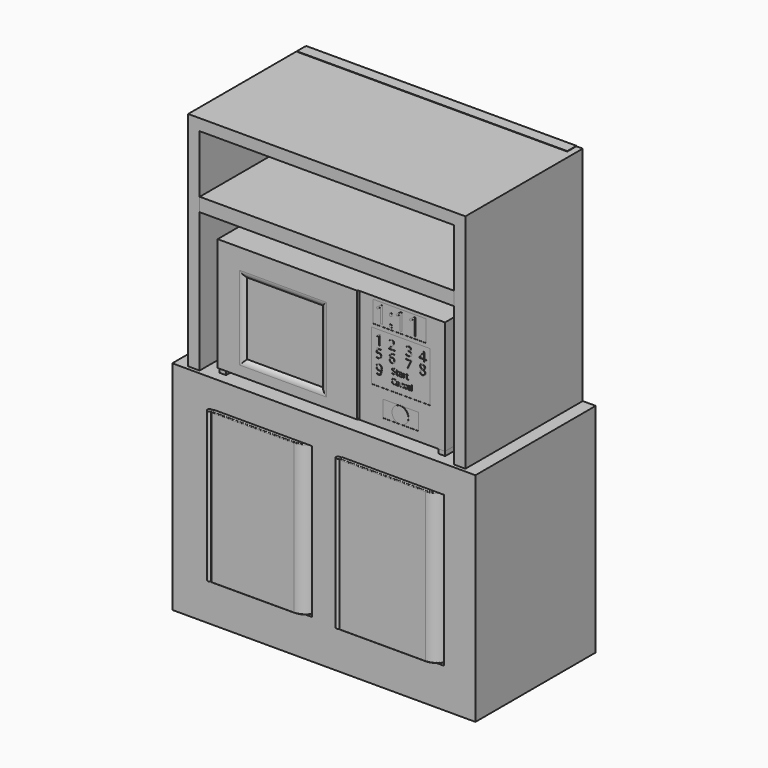
from build123d import *

# Parameters (mm, degrees)
F1_DEPTH        = 50.8
F2_DEPTH        = 52.07
F3_W            = 3.9822123945
F3_H            = 77.1151632071
F4_DEPTH        = 55.118
F5_DEPTH        = 38.354
F6_W            = 35.2624859661
F6_H            = 52.127157338
F6_W_2          = 33.9852
F7_DEPTH        = 43.18
F8_W            = 45.6940376786
F8_H            = 2.6725903153
F8_W_2          = 33.9852
F9_DEPTH        = 40.64
F10_R           = 2.8255137631
F11_DEPTH       = 25.4
F13_START       = 2.286
F12_W           = 78.4899894114
F12_H           = 39.2950200476
F12_R           = 2.8255137631
F13_DEPTH       = 42.418
F14_R           = 2.8255137631
F15_DEPTH       = 0.0762
F15_DEPTH_BACK  = 42.7228
F16_W           = 26.2017082423
F16_H           = 24.9313246459
F17_DEPTH       = 0.3048
F16_W_2         = 0.4919990897
F16_H_2         = 39.1533517959
F18_DEPTH       = 2.8702
F19_DEPTH       = 0.635
F20_T1_DEPTH    = 24.9313246459
F20_T3_DEPTH    = 26.2017082423
F20_T9_DEPTH    = 31.1330873344
F20_T13_DEPTH   = 29.862703738
F20_T20_DEPTH   = 29.862703738
F20_T24_DEPTH   = 31.1330873344
F20_T31_DEPTH   = 31.1330873344
F20_T35_DEPTH   = 29.862703738
F20_T42_DEPTH   = 31.1330873344
F20_T46_DEPTH   = 29.862703738
F21_W           = 18.2726848871
F21_H           = 7.4134916067
F21_W_2         = 20.2405880716
F21_H_2         = 17.3329468817
F21_W_3         = 12.3210083693
F21_H_3         = 5.7428432629
F21_R           = 2.8255137631
F15_FACE_R      = 2.8255137631
F22_DEPTH       = 0.0508
F23_TEXT_SIZE   = 4.6472272111
F23_TEXT_SIZE_2 = 4.3617124602
F23_TEXT_SIZE_3 = 4.3842428144
F23_TEXT_SIZE_4 = 2.6675458584
F23_TEXT_SIZE_5 = 2.4056812334
F23_TEXT_SIZE_6 = 4.3257706509
F23_TEXT_SIZE_7 = 4.6672040804
F23_TEXT_SIZE_8 = 4.7208482607
F24_DEPTH       = 0.127
F25_R           = 0.8497114132
F26_DEPTH       = 29.21
F27_W           = 33.685291186
F27_H           = 14.8179726675
F27_H_2         = 2.6725903153
F28_DEPTH       = 3.81
F27_W_2         = 34.7396545112
F27_H_3         = 52.0917661488
F29_DEPTH       = 3.81
F30_T1_DEPTH    = 76.6830152699
F30_2_T1_DEPTH  = 76.6852103972
F31_R           = 0.254
F31_2_R         = 0.254
F32_TEXT_SIZE   = 8.062650967
F33_DEPTH       = 0.0762
F35_START       = -9.652
F34_R           = 0.8068869831
F34_R_2         = 0.7608241077
F35_DEPTH       = 51.816
F37_DEPTH       = 2.1844
F38_R           = 0.1742456075
F38_W           = 0.127
F38_H           = 0.7986426353
F38_W_2         = 0.1268871129
F39_DEPTH       = 1.1684
F40_R           = 0.127
F41_R           = 0.0254
F42_W           = 2.2606
F42_H           = 1.7440778902
F42_W_2         = 2.2516623139
F42_H_2         = 1.757984166
F43_DEPTH       = 44.45
F44_W           = 88.0871986938
F44_H           = 4.7152489424
F45_DEPTH       = 46.7614


# Not quite as in the source:
# - a fillet or chamfer that OpenCascade refuses, or shapes differently, is made with other operations: its cross-section is extruded or revolved along the edge and cut away or added
# - a feature names something its author has since deleted; it is built from what else it names
# - Text() gives the source's letters only with a copy of the font that has no kerning and outlines rounded to 1/6400 em; it was checked with that copy


with BuildPart() as f1:
    # F0 (on Front) → F1 (new body)
    with BuildSketch(Plane.XZ):
        Polygon((57.3023967445, 76.9620016217), (-38.7095995247, 76.9620016217), (-38.7095995247, 0), (-34.7471995247, 0), (-34.7471995247, 72.9995965958), (53.3399991691, 72.9995965958), (53.3399991691, 0), (57.3023967445, 0), align=None)
    extrude(amount=F1_DEPTH)

    # F0 (on Front) → F2 (join)
    with BuildSketch(Plane.XZ):
        Polygon((-34.7471995247, 0), (-38.7095995247, 0), (-43.196324259, 0), (-43.196324259, -75.2101317048), (61.7981967445, -75.2101317048), (61.7981967445, 0), (57.3023967445, 0), (53.3399991691, 0), align=None)
    extrude(amount=F2_DEPTH)

    # F3 (on Right) → F4 (join)
    with BuildSketch(Plane.YZ):
        with Locations((-1.9911061972, 38.5575816035)):
            Rectangle(F3_W, F3_H)
    extrude(amount=F4_DEPTH)

    # F3 (on Right) → F5 (join)
    with BuildSketch(Plane.YZ):
        with Locations((-1.9911061972, 38.5575816035)):
            Rectangle(F3_W, F3_H)
    extrude(amount=-F5_DEPTH)

    # F6 (on face) → F7 (cut)
    with BuildSketch(Plane.XZ.offset(52.07)):
        with Locations((33.2693913952, -35.5714834295)):
            Rectangle(F6_W, F6_H)
        with Locations((-11.8306509047, -35.5714834295)):
            Rectangle(F6_W_2, F6_H)
    extrude(amount=-F7_DEPTH, mode=Mode.SUBTRACT)

    # F8 (on face) → F9 (join)
    with BuildSketch(Plane.XZ.offset(8.89)):
        Polygon((50.855986774, -39.7957935929), (5.1619490953, -39.7957935929), (5.1619490953, -44.7080158313), (50.855986774, -45.0032800436), align=None)
        Polygon((5.1619490953, -44.7080158313), (5.1619490953, -39.7957935929), (-28.8232509047, -39.7957935929), (-28.8232509047, -44.4884113967), align=None)
        with Locations((28.0089679346, -25.6614517421)):
            Rectangle(F8_W, F8_H)
        with Locations((-11.8306509047, -25.6614517421)):
            Rectangle(F8_W_2, F8_H)
    extrude(amount=F9_DEPTH)

    # F10 (on face) → F11 (cut)
    with BuildSketch(Plane.XZ.offset(3.9822123945)):
        with Locations((33.057577908, 7.6482067816)):
            Circle(F10_R)
    extrude(amount=-F11_DEPTH, mode=Mode.SUBTRACT)

    # F34 (on Top) → F35 (join)
    with BuildSketch(Plane.XY.offset(F35_START)):
        with Locations((-29.6579673886, -52.6868924499)):
            Circle(F34_R)
        with Locations((14.8290852085, -52.6868924499)):
            Circle(F34_R_2)
    extrude(amount=-F35_DEPTH)



with BuildPart() as f13:
    # F12 (on face) → F13 (new body)
    with BuildSketch(Plane.XZ.offset(3.9822123945).offset(F13_START)):
        with Locations((9.2983951809, 21.2607223075)):
            Rectangle(F12_W, F12_H)
        with Locations((33.057577908, 7.6482067816)):
            Circle(F12_R, mode=Mode.SUBTRACT)
    extrude(amount=F13_DEPTH)

    # F14 (on face) → F15 (join, two sides)
    with BuildSketch(Plane.XZ.offset(48.6862123945)) as f15_sk:
        with Locations((33.057577908, 7.6482067816)):
            Circle(F14_R)
    extrude(amount=F15_DEPTH)
    extrude(f15_sk.sketch, amount=-F15_DEPTH_BACK)

    # F16 (on face) → F17 (join)
    with BuildSketch(Plane.XZ.offset(48.6862123945)):
        Polygon((18.3940324932, 40.8427640796), (18.3940324932, 40.9082323313), (-29.9465995247, 40.9082323313), (-29.9465995247, 1.6132122837), (18.3940324932, 1.6132122837), (18.3940324932, 1.6894122837), align=None)
        with Locations((-7.3477765545, 19.4301092997)):
            Rectangle(F16_W, F16_H, mode=Mode.SUBTRACT)
    extrude(amount=F17_DEPTH)

    # F16 (on face) → F18 (cut)
    with BuildSketch(Plane.XZ.offset(48.6862123945)):
        with Locations((18.6400320381, 21.2660881816)):
            Rectangle(F16_W_2, F16_H_2)
    extrude(amount=-F18_DEPTH, mode=Mode.SUBTRACT)

    # F16 (on face) → F19 (cut)
    with BuildSketch(Plane.XZ.offset(48.6862123945)):
        with Locations((-7.3477765545, 19.4301092997)):
            Rectangle(F16_W, F16_H)
    extrude(amount=-F19_DEPTH, mode=Mode.SUBTRACT)

    # F20: fillet of radius 2.54 on 4 edges, made by hand

    # F20_s2 → F20_t1 (cut)
    with BuildSketch(Plane.XY.offset(6.9644469768)):
        with BuildLine():
            ThreePointArc((7.7256292035, -48.9910123945), (6.6331338945, -48.7440570953), (5.7530775666, -48.0512123945))
            Line((5.7530775666, -48.0512123945), (5.7530775666, -48.9910123945))
            Line((5.7530775666, -48.9910123945), (7.7256292035, -48.9910123945))
        make_face()
        with BuildLine():
            ThreePointArc((-22.4211823125, -48.9910123945), (-21.3286870036, -48.7440570953), (-20.4486306757, -48.0512123945))
            Line((-20.4486306757, -48.0512123945), (-20.4486306757, -48.9910123945))
            Line((-20.4486306757, -48.9910123945), (-22.4211823125, -48.9910123945))
        make_face()
    extrude(amount=F20_T1_DEPTH, mode=Mode.SUBTRACT)

    # F20_s4 → F20_t3 (cut)
    with BuildSketch(Plane.YZ.offset(-20.4486306757)):
        with BuildLine():
            ThreePointArc((-48.9910123945, 33.8683232595), (-48.7440570953, 32.7758279506), (-48.0512123945, 31.8957716227))
            Line((-48.0512123945, 31.8957716227), (-48.9910123945, 31.8957716227))
            Line((-48.9910123945, 31.8957716227), (-48.9910123945, 33.8683232595))
        make_face()
        with BuildLine():
            ThreePointArc((-48.9910123945, 4.9918953399), (-48.7440570953, 6.0843906489), (-48.0512123945, 6.9644469768))
            Line((-48.0512123945, 6.9644469768), (-48.9910123945, 6.9644469768))
            Line((-48.9910123945, 6.9644469768), (-48.9910123945, 4.9918953399))
        make_face()
    extrude(amount=F20_T3_DEPTH, mode=Mode.SUBTRACT)


with BuildPart() as f20_tool7:
    # F20_s8 → F20_t9 (new body)
    with BuildSketch(Plane.YZ.offset(-20.4486306757)):
        with BuildLine():
            ThreePointArc((-48.9910123945, 33.8683232595), (-48.7440570953, 32.7758279506), (-48.0512123945, 31.8957716227))
            Line((-48.0512123945, 31.8957716227), (-48.9910123945, 31.8957716227))
            Line((-48.9910123945, 31.8957716227), (-48.9910123945, 33.8683232595))
        make_face()
    extrude(amount=F20_T9_DEPTH)

    split(bisect_by=Plane.YZ.offset(5.7530775666), keep=Keep.TOP)


with BuildPart() as f20_tool11:
    # F20_s12 → F20_t13 (new body)
    with BuildSketch(Plane.XY.offset(36.8271507148)):
        with BuildLine():
            ThreePointArc((7.7256292035, -48.9910123945), (6.6331338945, -48.7440570953), (5.7530775666, -48.0512123945))
            Line((5.7530775666, -48.0512123945), (5.7530775666, -48.9910123945))
            Line((5.7530775666, -48.9910123945), (7.7256292035, -48.9910123945))
        make_face()
    extrude(amount=-F20_T13_DEPTH)

    split(bisect_by=Plane.XY.offset(31.8957716227), keep=Keep.TOP)


with BuildPart() as f20_tool7_1:
    add(f20_tool7.part)

    # F20_t15: intersect F20_tool11
    add(f20_tool11.part, mode=Mode.INTERSECT)


with BuildPart() as f13_1:
    add(f13.part)

    # F20_t5: cut F20_tool7
    add(f20_tool7_1.part, mode=Mode.SUBTRACT)


with BuildPart() as f20_tool18:
    # F20_s19 → F20_t20 (new body)
    with BuildSketch(Plane.XY.offset(31.8957716227)):
        with BuildLine():
            ThreePointArc((7.7256292035, -48.9910123945), (6.6331338945, -48.7440570953), (5.7530775666, -48.0512123945))
            Line((5.7530775666, -48.0512123945), (5.7530775666, -48.9910123945))
            Line((5.7530775666, -48.9910123945), (7.7256292035, -48.9910123945))
        make_face()
    extrude(amount=-F20_T20_DEPTH)

    split(bisect_by=Plane.XY.offset(6.9644469768), keep=Keep.BOTTOM)


with BuildPart() as f20_tool22:
    # F20_s23 → F20_t24 (new body)
    with BuildSketch(Plane.YZ.offset(10.6844566587)):
        with BuildLine():
            ThreePointArc((-48.9910123945, 4.9918953399), (-48.7440570953, 6.0843906489), (-48.0512123945, 6.9644469768))
            Line((-48.0512123945, 6.9644469768), (-48.9910123945, 6.9644469768))
            Line((-48.9910123945, 6.9644469768), (-48.9910123945, 4.9918953399))
        make_face()
    extrude(amount=-F20_T24_DEPTH)

    split(bisect_by=Plane.YZ.offset(5.7530775666), keep=Keep.TOP)


with BuildPart() as f20_tool18_1:
    add(f20_tool18.part)

    # F20_t26: intersect F20_tool22
    add(f20_tool22.part, mode=Mode.INTERSECT)


with BuildPart() as f13_2:
    add(f13_1.part)

    # F20_t16: cut F20_tool18
    add(f20_tool18_1.part, mode=Mode.SUBTRACT)


with BuildPart() as f20_tool29:
    # F20_s30 → F20_t31 (new body)
    with BuildSketch(Plane.YZ.offset(-25.3800097678)):
        with BuildLine():
            ThreePointArc((-48.9910123945, 33.8683232595), (-48.7440570953, 32.7758279506), (-48.0512123945, 31.8957716227))
            Line((-48.0512123945, 31.8957716227), (-48.9910123945, 31.8957716227))
            Line((-48.9910123945, 31.8957716227), (-48.9910123945, 33.8683232595))
        make_face()
    extrude(amount=F20_T31_DEPTH)

    split(bisect_by=Plane.YZ.offset(-20.4486306757), keep=Keep.BOTTOM)


with BuildPart() as f20_tool33:
    # F20_s34 → F20_t35 (new body)
    with BuildSketch(Plane.XY.offset(6.9644469768)):
        with BuildLine():
            ThreePointArc((-22.4211823125, -48.9910123945), (-21.3286870036, -48.7440570953), (-20.4486306757, -48.0512123945))
            Line((-20.4486306757, -48.0512123945), (-20.4486306757, -48.9910123945))
            Line((-20.4486306757, -48.9910123945), (-22.4211823125, -48.9910123945))
        make_face()
    extrude(amount=F20_T35_DEPTH)

    split(bisect_by=Plane.XY.offset(31.8957716227), keep=Keep.TOP)


with BuildPart() as f20_tool29_1:
    add(f20_tool29.part)

    # F20_t37: intersect F20_tool33
    add(f20_tool33.part, mode=Mode.INTERSECT)


with BuildPart() as f13_3:
    add(f13_2.part)

    # F20_t27: cut F20_tool29
    add(f20_tool29_1.part, mode=Mode.SUBTRACT)


with BuildPart() as f20_tool40:
    # F20_s41 → F20_t42 (new body)
    with BuildSketch(Plane.YZ.offset(5.7530775666)):
        with BuildLine():
            ThreePointArc((-48.9910123945, 4.9918953399), (-48.7440570953, 6.0843906489), (-48.0512123945, 6.9644469768))
            Line((-48.0512123945, 6.9644469768), (-48.9910123945, 6.9644469768))
            Line((-48.9910123945, 6.9644469768), (-48.9910123945, 4.9918953399))
        make_face()
    extrude(amount=-F20_T42_DEPTH)

    split(bisect_by=Plane.YZ.offset(-20.4486306757), keep=Keep.BOTTOM)


with BuildPart() as f20_tool44:
    # F20_s45 → F20_t46 (new body)
    with BuildSketch(Plane.XY.offset(2.0330678847)):
        with BuildLine():
            ThreePointArc((-22.4211823125, -48.9910123945), (-21.3286870036, -48.7440570953), (-20.4486306757, -48.0512123945))
            Line((-20.4486306757, -48.0512123945), (-20.4486306757, -48.9910123945))
            Line((-20.4486306757, -48.9910123945), (-22.4211823125, -48.9910123945))
        make_face()
    extrude(amount=F20_T46_DEPTH)

    split(bisect_by=Plane.XY.offset(6.9644469768), keep=Keep.BOTTOM)


with BuildPart() as f20_tool40_1:
    add(f20_tool40.part)

    # F20_t48: intersect F20_tool44
    add(f20_tool44.part, mode=Mode.INTERSECT)


with BuildPart() as f13_4:
    add(f13_3.part)

    # F20_t38: cut F20_tool40
    add(f20_tool40_1.part, mode=Mode.SUBTRACT)

    # F21 (on face) + F15_face (on face) → F22 (cut)
    with BuildSketch(Plane.XZ.offset(48.6862123945)):
        with Locations((32.752885604, 36.1756414401)):
            Rectangle(F21_W, F21_H)
        with Locations((33.1727000142, 22.5801277634)):
            Rectangle(F21_W_2, F21_H_2)
        with Locations((33.1698926166, 7.6576885767)):
            Rectangle(F21_W_3, F21_H_3)
        with Locations((33.057577908, 7.6482067816)):
            Circle(F21_R, mode=Mode.SUBTRACT)
    with BuildSketch(Plane(origin=(33.057577908, -48.7624123945, 7.6482067816), x_dir=(1, 0, 0), z_dir=(0, -1, 0))):
        Circle(F15_FACE_R)
    extrude(amount=-F22_DEPTH, mode=Mode.SUBTRACT)

    # F23 (on face) → F24 (cut)
    with BuildSketch(Plane.XZ.offset(48.6354123945)):
        with Locations((24.4673758674, 26.5110091874)):
            Text('1', F23_TEXT_SIZE, font='Open Sans', text_align=(TextAlign.LEFT, TextAlign.BOTTOM))
        with Locations((28.9693809518, 26.5110091874)):
            Text('2', F23_TEXT_SIZE_2, font='Open Sans', text_align=(TextAlign.LEFT, TextAlign.BOTTOM))
        with Locations((34.8159538121, 26.4947873323)):
            Text('3', F23_TEXT_SIZE_3, font='Open Sans', text_align=(TextAlign.LEFT, TextAlign.BOTTOM))
        with Locations((39.6293903202, 26.4947873323)):
            Text('4', F23_TEXT_SIZE_3, font='Open Sans', text_align=(TextAlign.LEFT, TextAlign.BOTTOM))
        with Locations((30.0131645054, 19.2666854709)):
            Text('Start', F23_TEXT_SIZE_4, font='Open Sans', text_align=(TextAlign.LEFT, TextAlign.BOTTOM))
        with Locations((29.9500077963, 16.2383075804)):
            Text('Cancel', F23_TEXT_SIZE_5, font='Open Sans', text_align=(TextAlign.LEFT, TextAlign.BOTTOM))
        with Locations((24.4673758674, 22.4644691564)):
            Text('5', F23_TEXT_SIZE_6, font='Open Sans', text_align=(TextAlign.LEFT, TextAlign.BOTTOM))
        with Locations((28.9693809518, 22.4644691564)):
            Text('6', F23_TEXT_SIZE_6, font='Open Sans', text_align=(TextAlign.LEFT, TextAlign.BOTTOM))
        with Locations((34.8159538121, 22.4644691564)):
            Text('7', F23_TEXT_SIZE_6, font='Open Sans', text_align=(TextAlign.LEFT, TextAlign.BOTTOM))
        with Locations((39.5429395139, 22.2836155444)):
            Text('8', F23_TEXT_SIZE_7, font='Open Sans', text_align=(TextAlign.LEFT, TextAlign.BOTTOM))
        with Locations((24.4673758674, 17.4941010773)):
            Text('9', F23_TEXT_SIZE_8, font='Open Sans', text_align=(TextAlign.LEFT, TextAlign.BOTTOM))
    extrude(amount=-F24_DEPTH, mode=Mode.SUBTRACT)

    # F25 (on face) → F26 (join)
    with BuildSketch(Plane(origin=(0, -5.9634123945, 0), x_dir=(-1, 0, 0), z_dir=(0, 1, 0))):
        with Locations((-33.057577908, 7.6482067816)):
            Circle(F25_R)
    extrude(amount=F26_DEPTH)

    # F32 (on face) → F33 (join)
    with BuildSketch(Plane.XZ.offset(48.6354123945)):
        with Locations((24.0707267076, 33.2496277988)):
            Text('1:11', F32_TEXT_SIZE, font='Open Sans', text_align=(TextAlign.LEFT, TextAlign.BOTTOM))
    extrude(amount=F33_DEPTH)

    # F36 (on face) → F37 (join)
    with BuildSketch(Plane(origin=(0, 23.2465876055, 0), x_dir=(-1, 0, 0), z_dir=(0, 1, 0))):
        with BuildLine():
            Line((-32.0737659931, 8.3758132532), (-32.6187176704, 8.3758132532))
            ThreePointArc((-32.6187176704, 8.3758132532), (-32.317674523, 8.0660015476), (-32.2078664948, 7.6482067816))
            ThreePointArc((-32.2078664948, 7.6482067816), (-32.3147240321, 7.2356808979), (-32.6084203819, 6.9269114174))
            Line((-32.6084203819, 6.9269114174), (-32.0737659931, 6.9269114174))
            Line((-32.0737659931, 6.9269114174), (-32.0737659931, 8.3758132532))
        make_face()
        with BuildLine():
            Line((-32.6187176704, 8.3758132532), (-33.4964381457, 8.3758132532))
            ThreePointArc((-33.4964381457, 8.3758132532), (-33.9072678631, 7.6542454948), (-33.5067354342, 6.9269114174))
            Line((-33.5067354342, 6.9269114174), (-32.6084203819, 6.9269114174))
            ThreePointArc((-32.6084203819, 6.9269114174), (-32.3147240321, 7.2356808979), (-32.2078664948, 7.6482067816))
            ThreePointArc((-32.2078664948, 7.6482067816), (-32.317674523, 8.0660015476), (-32.6187176704, 8.3758132532))
        make_face()
        with BuildLine():
            Line((-33.4964381457, 8.3758132532), (-34.0495407581, 8.3758132532))
            Line((-34.0495407581, 8.3758132532), (-34.0495407581, 6.9269114174))
            Line((-34.0495407581, 6.9269114174), (-33.5067354342, 6.9269114174))
            ThreePointArc((-33.5067354342, 6.9269114174), (-33.9072678631, 7.6542454948), (-33.4964381457, 8.3758132532))
        make_face()
    extrude(amount=F37_DEPTH)

    # F38 (on face) → F39 (join)
    with BuildSketch(Plane(origin=(0, 25.4309876055, 0), x_dir=(-1, 0, 0), z_dir=(0, 1, 0))):
        with Locations((-33.0648608506, 8.0952914432)):
            Circle(F38_R)
        with Locations((-32.6356267502, 7.5019067153)):
            Rectangle(F38_W, F38_H)
        with Locations((-33.4853763225, 7.5019067153)):
            Rectangle(F38_W_2, F38_H)
    extrude(amount=F39_DEPTH)

    # F40
    f40_edges = [f13_4.edges().sort_by_distance(p)[0] for p in [
        (33.239106, 26.599388, 8.095291),
    ]]
    fillet(f40_edges, radius=F40_R)

    # F41
    f41_edges = [f13_4.edges().sort_by_distance(p)[0] for p in [
        (33.421933, 26.599388, 7.501907),
        (33.54882, 26.599388, 7.501907),
        (33.485376, 26.599388, 7.102585),
        (33.485376, 26.599388, 7.901228),
        (32.635627, 26.599388, 7.901228),
        (32.699127, 26.599388, 7.501907),
        (32.635627, 26.599388, 7.102585),
        (32.572127, 26.599388, 7.501907),
    ]]
    fillet(f41_edges, radius=F41_R)


with BuildPart() as f28:
    # F27 (on face) → F28 (new body)
    with BuildSketch(Plane.XZ.offset(49.53)):
        Polygon((4.8620402813, -26.9977468997), (-28.8232509047, -26.9977468997), (-28.8232509047, -61.6335980594), (4.8620402813, -61.5967549384), align=None)
        with Locations((-11.9806053117, -16.9161702506)):
            Rectangle(F27_W, F27_H)
        with Locations((-11.9806053117, -25.6614517421)):
            Rectangle(F27_W, F27_H_2)
    extrude(amount=F28_DEPTH)

    # F30: fillet of radius 5.08 on 1 edges, made by hand

    # F30_s2 → F30_t1 (cut)
    with BuildSketch(Plane.XY.offset(-73.8934770626)):
        with BuildLine():
            ThreePointArc((4.8620402813, -49.53), (3.0542034049, -52.2760926284), (-0.0566485684, -53.34))
            Line((-0.0566485684, -53.34), (4.8620402813, -53.34))
            Line((4.8620402813, -53.34), (4.8620402813, -49.53))
        make_face()
    extrude(amount=F30_T1_DEPTH, mode=Mode.SUBTRACT)

    # F31
    f31_edges = [f28.edges().sort_by_distance(p)[0] for p in [
        (-14.43995, -53.34, -9.507184),
        (-28.823251, -53.34, -35.570391),
        (-14.43995, -53.34, -61.617866),
        (3.054203, -52.276093, -61.598732),
    ]]
    fillet(f31_edges, radius=F31_R)


with BuildPart() as f29:
    # F27 (on face) → F29 (new body)
    with BuildSketch(Plane.XZ.offset(49.53)):
        with Locations((33.0074708909, -35.550871864)):
            Rectangle(F27_W_2, F27_H_3)
    extrude(amount=F29_DEPTH)

    # F30#2: fillet of radius 5.08 on 1 edges, made by hand

    # F30_2_s2 → F30_2_t1 (cut)
    with BuildSketch(Plane.XY.offset(-73.8934770626)):
        with BuildLine():
            ThreePointArc((50.3772981465, -49.53), (48.5694612701, -52.2760926284), (45.4586092968, -53.34))
            Line((45.4586092968, -53.34), (50.3772981465, -53.34))
            Line((50.3772981465, -53.34), (50.3772981465, -49.53))
        make_face()
    extrude(amount=F30_2_T1_DEPTH, mode=Mode.SUBTRACT)

    # F31#2
    f31_2_edges = [f29.edges().sort_by_distance(p)[0] for p in [
        (30.548126, -53.34, -9.504989),
        (45.458609, -53.34, -35.550872),
        (30.548126, -53.34, -61.596755),
        (15.637644, -53.34, -35.550872),
        (48.569461, -52.276093, -9.504989),
        (48.569461, -52.276093, -61.596755),
    ]]
    fillet(f31_2_edges, radius=F31_2_R)


with BuildPart() as f1_1:
    add(f1.part)

    add(f13_4.part)  # F43 merges F13
    # F42 (on face) → F43 (join)
    with BuildSketch(Plane.XZ.offset(3.9822123945)):
        with Locations((-28.6055185053, 0.8720389451)):
            Rectangle(F42_W, F42_H)
        with Locations((47.2890995443, 0.878992083)):
            Rectangle(F42_W_2, F42_H_2)
    extrude(amount=F43_DEPTH)

    # F44 (on face) → F45 (join)
    with BuildSketch(Plane.XZ.offset(3.9822123945)):
        with Locations((9.2963998222, 50.6189726293)):
            Rectangle(F44_W, F44_H)
    extrude(amount=F45_DEPTH)


solid = Compound([f28.part, f29.part, f1_1.part])
